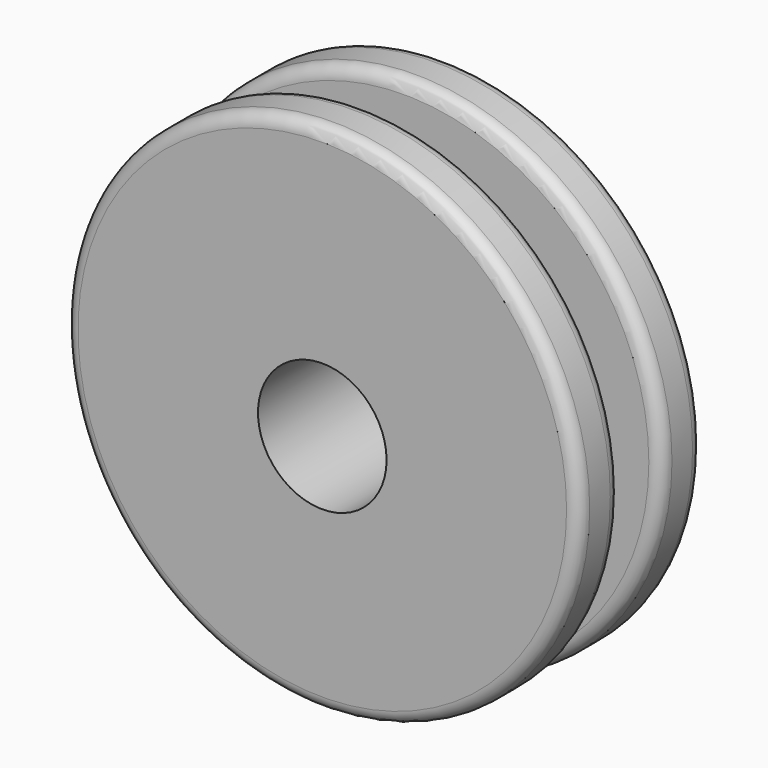
from build123d import *

# Parameters (mm, degrees)
F0_R     = 100
F1_DEPTH = 20
F2_R     = 60
F3_DEPTH = 20
F4_R     = 100
F5_DEPTH = 20
F6_R     = 25
F7_DEPTH = 100
F8_R     = 5


with BuildPart() as f1:
    # F0 (on Front) → F1 (new body)
    with BuildSketch(Plane.XZ):
        Circle(F0_R)
    extrude(amount=F1_DEPTH)

    # F2 (on face) → F3 (join)
    with BuildSketch(Plane.XZ.offset(20)):
        Circle(F2_R)
    extrude(amount=F3_DEPTH)

    # F4 (on face) → F5 (join)
    with BuildSketch(Plane.XZ.offset(40)):
        Circle(F4_R)
    extrude(amount=F5_DEPTH)

    # F6 (on face) → F7 (cut)
    with BuildSketch(Plane.XZ.offset(60)):
        with Locations((0, -5.704428)):
            Circle(F6_R)
    extrude(amount=-F7_DEPTH, mode=Mode.SUBTRACT)

    # F8
    f8_edges = [f1.edges().sort_by_distance(p)[0] for p in [
        (-100, -60, 0),
        (-100, -40, 0),
        (-100, -20, 0),
        (-100, 0, 0),
    ]]
    fillet(f8_edges, radius=F8_R)


solid = f1.part
